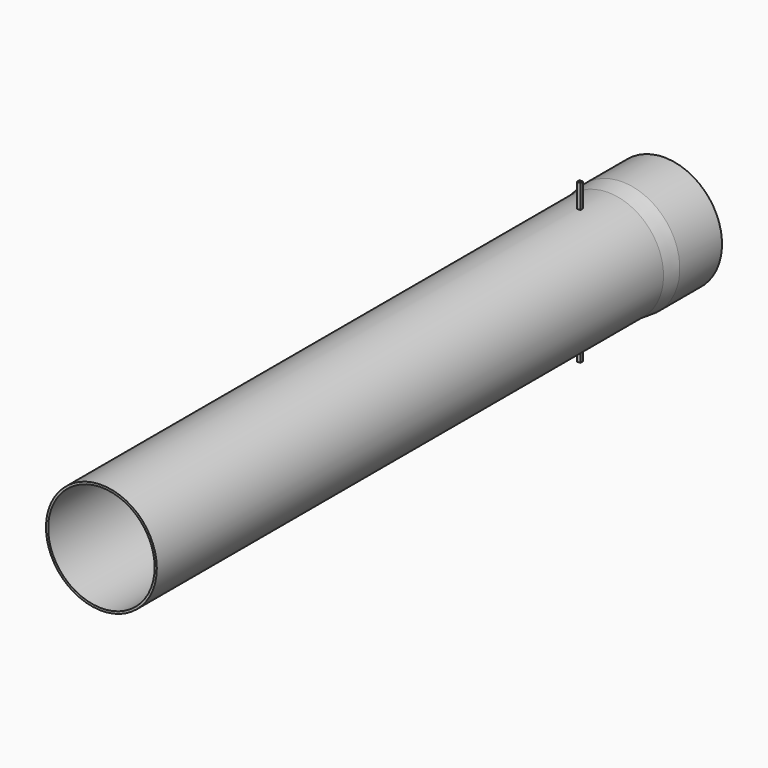
from build123d import *

# Parameters (mm, degrees)
F0_R        = 157.5
F1_DEPTH    = 1800
F3_R        = 163.7
F1_FACE_R   = 157.5
F5_DEPTH    = 150
F6_T        = 6.2
F6_T4_ANGLE = 180.000000001
F6_T6_ANGLE = 180.000000001
F7_W        = 10
F7_H        = 10
F8_DEPTH    = 350
F9_DEPTH    = 225
F10_T       = -1
F11_W       = 10
F11_H       = 35
F12_DEPTH   = 2
F13_D       = 5.5
F14_D       = 5.5


# Not quite as in the source:
# - a shell that OpenCascade refuses in one call is made with other operations: the cavity is built on its own and cut out
# - a feature names something its author has since deleted; it is built from what else it names


with BuildPart() as f1:
    # F0 (on Front) → F1 (new body)
    with BuildSketch(Plane.XZ):
        Circle(F0_R)
    extrude(amount=F1_DEPTH)

    # F3 (on offset) → F4 section 0
    with BuildSketch(Plane(origin=(0, 50, 0), x_dir=(-1, 0, 0), z_dir=(0, 1, 0))):
        Circle(F3_R)
    # F1_face (on face) → F4 section 1
    with BuildSketch(Plane(origin=(0, 0, 0), x_dir=(1, 0, 0), z_dir=(0, 1, 0))):
        Circle(F1_FACE_R)
    loft()

    # F5 (add): a face of the model
    f5_faces = [f1.faces().sort_by_distance(p)[0] for p in [
        (0, 50, 0),
    ]]
    extrude(f5_faces, amount=F5_DEPTH)

    # F6: shell of thickness 6.2, made by hand


with BuildPart() as f6_core1:
    # F6_t2: copy of F1
    add(f1.part)

    # the walls: a layer under each face that stays
    f6_faces = [f6_core1.faces().sort_by_distance(p)[0] for p in [
        (-157.5, -900, 0),
        (160.6, 25, 0),
        (163.7, 125, 0),
    ]]
    thicken(f6_faces, amount=-F6_T, mode=Mode.SUBTRACT)

    # F6_s3 → F6_t4 (revolve, cut)
    with BuildSketch(Plane.XY):
        Polygon((157.6235287713, -0.0076295676), (151.3, 0), (151.3, 0.3829336184), (151.3471228701, 0.7629567641), align=None)
    revolve(axis=Axis((0, 0, 0), (0, -1, 0)), revolution_arc=F6_T4_ANGLE, mode=Mode.SUBTRACT)

    # F6_s5 → F6_t6 (revolve, cut)
    with BuildSketch(Plane.XY):
        Polygon((-157.6235287713, -0.0076295676), (-151.3, 0), (-151.3, 0.3829336184), (-151.3471228701, 0.7629567641), align=None)
    revolve(axis=Axis((0, 0, 0), (0, -1, 0)), revolution_arc=F6_T6_ANGLE, mode=Mode.SUBTRACT)


with BuildPart() as f1_1:
    add(f1.part)

    # what is left inside the walls is the cavity
    f6_cavity = [f6_core1.part.solids().sort_by_distance(p)[0] for p in [
        (-151.238, -1199.872355, 0),
    ]]
    add(f6_cavity, mode=Mode.SUBTRACT)

    # F7 (on Top) → F8 (cut, symmetric)
    with BuildSketch(Plane.XY):
        with Locations((0, -100)):
            Rectangle(F7_W, F7_H)
    extrude(amount=F8_DEPTH, both=True, mode=Mode.SUBTRACT)


with BuildPart() as f9:
    # F7 (on Top) → F9 (new body, symmetric)
    with BuildSketch(Plane.XY):
        with Locations((0, -100)):
            Rectangle(F7_W, F7_H)
    extrude(amount=F9_DEPTH, both=True)

    # F10
    f10_openings = [f9.faces().sort_by_distance(p)[0] for p in [
        (0, -100, 225),
        (0, -100, -225),
    ]]
    offset(amount=F10_T, openings=f10_openings)

    # F13 (through all)
    with Locations(Plane.XZ.offset(105)):
        with Locations((0, -47.5), (0, -62.5)):
            Hole(F13_D / 2)


with BuildPart() as f12:
    # F11 (on face) → F12 (new body)
    with BuildSketch(Plane.XZ.offset(105)):
        with Locations((0, -55)):
            Rectangle(F11_W, F11_H)
    extrude(amount=F12_DEPTH)

    # F14 (through all)
    with Locations(Plane(origin=(0, -105, 0), x_dir=(1, 0, 0), z_dir=(0, 1, 0))):
        with Locations((0, 47.5), (0, 62.5)):
            Hole(F14_D / 2)


solid = Compound([f1_1.part, f9.part, f12.part])
